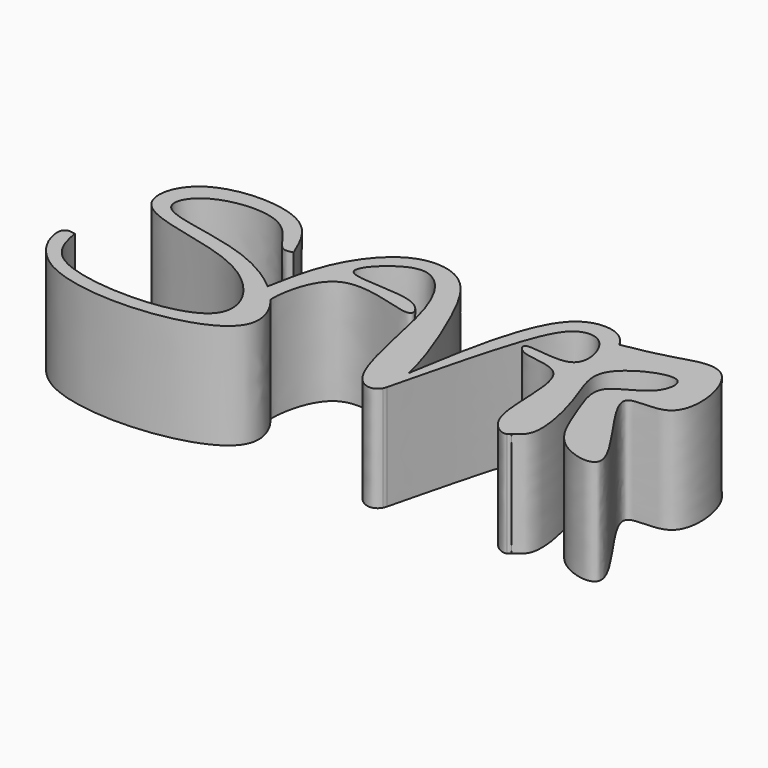
from build123d import *

# Parameters (mm, degrees)
F1_DEPTH = 25.4


# Not quite as in the source:
# - ends of sketch curves that miss each other by under 0.0002 mm in the source are joined


with BuildPart() as f1:
    # F0 (on Top) → F1 (new body)
    with BuildSketch(Plane.XY):
        with BuildLine():
            add(Edge.make_bspline(
                [(-24.6787276119, 32.8070372343), (-25.5273015557, 32.5405150057), (-28.1014851586, 31.7320089754), (-32.90699094, 43.9368654397), (-52.875406472, 41.759288149), (-57.7038976314, 29.1589085216), (-35.7015094106, 29.7052712427), (-22.4863598149, 21.2072316293), (-19.8319724851, 18.9303140968)],
                knots=[0, 0, 0, 0, 0.0470421865, 0.1427043876, 0.2659306317, 0.3432443836, 0.4950399565, 0.5430279559, 0.5430279559, 0.5430279559, 0.5430279559], degree=3))
            add(Edge.make_bspline(
                [(-24.6787276119, 32.8070372343), (-26.5064995292, 37.1770989066), (-30.6352734039, 47.0486787753), (-57.5475208508, 46.96673089), (-62.4266866267, 26.0189740304), (-28.0149183626, 26.4603141136), (-10.52810376, -1.8863198777), (-58.7127529187, -1.6477709858), (-60.8782500601, 8.9999767274), (-61.6968199611, 13.0248842761)],
                knots=[0, 0, 0, 0, 0.1202382283, 0.2716074424, 0.38221019, 0.5584756929, 0.6980251192, 0.8858518243, 1, 1, 1, 1], degree=3))
            add(Edge.make_bspline(
                [(-15.8314434419, 14.8124826193), (-12.8167424406, 10.9820745517), (-8.3770839751, -3.436383487), (-60.1878877743, -8.036598746), (-66.2173758507, 13.782419329), (-62.7256533774, 13.1972916958), (-61.6968199611, 13.0248842761)],
                knots=[0.5706803148, 0.5706803148, 0.5706803148, 0.5706803148, 0.6455092316, 0.8394088149, 0.9526819274, 1, 1, 1, 1], degree=3))
            add(Edge.make_bspline(
                [(-16.0199403512, 15.048879084), (-15.97340642, 14.8563692593), (-15.9033936949, 14.8336509493), (-15.8314434419, 14.8124826193)],
                knots=[0.9896211656, 0.9896211656, 0.9896211656, 0.9896211656, 1, 1, 1, 1], degree=3))
            add(Edge.make_bspline(
                [(-19.8319724851, 18.9303140968), (-18.387658044, 17.6913898312), (-17.0972678041, 16.3826850288), (-16.0199403512, 15.048879084)],
                knots=[0.5430279559, 0.5430279559, 0.5430279559, 0.5430279559, 0.5691393526, 0.5691393526, 0.5691393526, 0.5691393526], degree=3))
        make_face()
        with BuildLine():
            add(Edge.make_bspline(
                [(-19.8319724851, 18.9303140968), (-18.8344760031, 24.2294951854), (-16.8978653598, 34.5465657632), (-6.7743663409, 46.7500210317), (6.8605077442, 45.9638720477), (14.2191273717, 33.5824908681), (21.6696104289, 14.3933148786), (23.0455104144, 7.8380652192)],
                knots=[0, 0, 0, 0, 0.0756121009, 0.147274394, 0.2086812387, 0.2887345767, 0.3572017989, 0.3572017989, 0.3572017989, 0.3572017989], degree=3))
            add(Edge.make_bspline(
                [(-19.8319724851, 18.9303140968), (-18.387658044, 17.6913898312), (-17.0972678041, 16.3826850288), (-16.0199403512, 15.048879084)],
                knots=[0.5430279559, 0.5430279559, 0.5430279559, 0.5430279559, 0.5691393526, 0.5691393526, 0.5691393526, 0.5691393526], degree=3))
            add(Edge.make_bspline(
                [(23.1118220836, 0), (22.177252315, -1.7340239565), (14.5773230299, -1.6966887198), (11.0961627452, 28.9295857186), (3.7256594235, 41.5664043956), (-4.1210514113, 43.3103447304), (-17.5436302823, 30.2403774921), (5.7533981015, 33.779177956), (11.0421016778, 23.3480646444), (-14.612230045, 36.7399787183), (-16.3443080286, 16.3907808564), (-16.0199403512, 15.048879084)],
                knots=[0.393623583, 0.393623583, 0.393623583, 0.393623583, 0.4353913281, 0.5377331001, 0.609740231, 0.6592510214, 0.7193383912, 0.7960567893, 0.8361379212, 0.917274851, 0.9896211656, 0.9896211656, 0.9896211656, 0.9896211656], degree=3))
            add(Edge.make_bspline(
                [(23.4237621025, 0.8001007005), (23.3421922869, 0.5029517859), (23.2386923409, 0.2353982259), (23.1118220836, 0)],
                knots=[0.3879535039, 0.3879535039, 0.3879535039, 0.3879535039, 0.393623583, 0.393623583, 0.393623583, 0.393623583], degree=3))
            add(Edge.make_bspline(
                [(23.0455104144, 7.8380652192), (23.6634889039, 4.8938081328), (23.86615644, 2.4116894523), (23.4237621025, 0.8001007005)],
                knots=[0.3572017989, 0.3572017989, 0.3572017989, 0.3572017989, 0.3879535039, 0.3879535039, 0.3879535039, 0.3879535039], degree=3))
        make_face()
        with BuildLine():
            add(Edge.make_bspline(
                [(-16.0199403512, 15.048879084), (-15.97340642, 14.8563692593), (-15.9033936949, 14.8336509493), (-15.8314434419, 14.8124826193)],
                knots=[0.9896211656, 0.9896211656, 0.9896211656, 0.9896211656, 1, 1, 1, 1], degree=3))
            add(Edge.make_bspline(
                [(-16.0199403512, 15.048879084), (-15.9563619495, 14.9701646226), (-15.8935255947, 14.89136274), (-15.8314434419, 14.8124826193)],
                knots=[0.5691393526, 0.5691393526, 0.5691393526, 0.5691393526, 0.5706803148, 0.5706803148, 0.5706803148, 0.5706803148], degree=3))
        make_face()
        with BuildLine():
            add(Edge.make_bspline(
                [(23.0455104144, 7.8380652192), (24.4324002035, 16.2806044304), (26.8519423128, 31.2653069215), (33.7083031751, 46.5916934343), (43.5702899083, 46.203123325), (46.2558693347, 42.6872189335), (46.7942668802, 41.7043013302)],
                knots=[0, 0, 0, 0, 0.0922168762, 0.1637277559, 0.2200942558, 0.23759776, 0.23759776, 0.23759776, 0.23759776], degree=3))
            add(Edge.make_bspline(
                [(23.0455104144, 7.8380652192), (23.6634889039, 4.8938081328), (23.86615644, 2.4116894523), (23.4237621025, 0.8001007005)],
                knots=[0.3572017989, 0.3572017989, 0.3572017989, 0.3572017989, 0.3879535039, 0.3879535039, 0.3879535039, 0.3879535039], degree=3))
            add(Edge.make_bspline(
                [(53.0788488686, 0), (51.8984399331, -0.5129918214), (44.5848763075, 3.7283170523), (49.1362338719, 28.5544108949), (34.8165799276, 26.4831796905), (31.1780051516, 32.2004713219), (48.3201512021, 26.7229973916), (44.5678259808, 41.4874538831), (36.376462422, 42.3677304518), (30.6036182602, 31.4239322121), (24.2879136847, 3.9486155232), (23.4239237173, 0.8006904499), (23.4237621025, 0.8001007005)],
                knots=[0.4289942329, 0.4289942329, 0.4289942329, 0.4289942329, 0.4767021069, 0.5614775501, 0.6211663392, 0.6508244204, 0.7128544037, 0.7693222766, 0.8141842446, 0.8799646816, 0.9827832344, 0.9828025139, 0.9828025139, 0.9828025139, 0.9828025139], degree=3))
            add(Edge.make_bspline(
                [(53.6664426327, 0.63326415), (53.3590889397, 0.4114939862), (53.2189711295, 0.2057502607), (53.0788488686, 0)],
                knots=[0.9808770796, 0.9808770796, 0.9808770796, 0.9808770796, 1, 1, 1, 1], degree=3))
            add(Edge.make_bspline(
                [(46.7942668802, 41.7043013302), (48.6032933073, 38.4016786955), (50.3660101546, 25.8827463669), (53.5382364777, 8.1673975806), (54.0836898285, 1.5815416662), (53.6664426327, 0.63326415)],
                knots=[0.23759776, 0.23759776, 0.23759776, 0.23759776, 0.2964098812, 0.385024933, 0.4183512362, 0.4183512362, 0.4183512362, 0.4183512362], degree=3))
        make_face()
        with BuildLine():
            add(Edge.make_bspline(
                [(23.4237621025, 0.8001007005), (23.3421922869, 0.5029517859), (23.2386923409, 0.2353982259), (23.1118220836, 0)],
                knots=[0.3879535039, 0.3879535039, 0.3879535039, 0.3879535039, 0.393623583, 0.393623583, 0.393623583, 0.393623583], degree=3))
            add(Edge.make_bspline(
                [(23.4237621025, 0.8001007005), (23.2793710251, 0.2741020489), (23.2183930531, 0.1282770233), (23.1118220836, 0)],
                knots=[0.9828025139, 0.9828025139, 0.9828025139, 0.9828025139, 1, 1, 1, 1], degree=3))
        make_face()
        with BuildLine():
            add(Edge.make_bspline(
                [(46.7942668802, 41.7043013302), (50.3848090207, 42.3444269721), (57.5784609028, 43.6240432253), (71.8688709785, 49.2296239678), (76.4397987852, 22.0429179865), (52.8460197012, 29.7031437768), (81.6110286462, -1.4014680593), (62.3170902407, 1.8533546119), (58.0399247272, 14.7977347688), (52.7378625165, 26.9256595732), (65.0537492941, 29.5782405699), (66.4716848994, 40.8014290246), (47.9292406475, 32.4847086055), (54.1956479046, 20.498618098), (58.4414610746, 2.7191685618), (54.2851661425, 1.0797023003), (53.6664426327, 0.63326415)],
                knots=[0, 0, 0, 0, 0.0696168426, 0.139557473, 0.2251970613, 0.2894080935, 0.3920456325, 0.4510893761, 0.5301929119, 0.5963398453, 0.6612406867, 0.7111688526, 0.7855380932, 0.8574622076, 0.9423813637, 0.9808770796, 0.9808770796, 0.9808770796, 0.9808770796], degree=3))
            add(Edge.make_bspline(
                [(46.7942668802, 41.7043013302), (48.6032933073, 38.4016786955), (50.3660101546, 25.8827463669), (53.5382364777, 8.1673975806), (54.0836898285, 1.5815416662), (53.6664426327, 0.63326415)],
                knots=[0.23759776, 0.23759776, 0.23759776, 0.23759776, 0.2964098812, 0.385024933, 0.4183512362, 0.4183512362, 0.4183512362, 0.4183512362], degree=3))
        make_face()
        with BuildLine():
            add(Edge.make_bspline(
                [(53.6664426327, 0.63326415), (53.3590889397, 0.4114939862), (53.2189711295, 0.2057502607), (53.0788488686, 0)],
                knots=[0.9808770796, 0.9808770796, 0.9808770796, 0.9808770796, 1, 1, 1, 1], degree=3))
            add(Edge.make_bspline(
                [(53.6664426327, 0.63326415), (53.5331917132, 0.3304248446), (53.342182515, 0.1144417014), (53.0788488686, 0)],
                knots=[0.4183512362, 0.4183512362, 0.4183512362, 0.4183512362, 0.4289942329, 0.4289942329, 0.4289942329, 0.4289942329], degree=3))
        make_face()
    extrude(amount=F1_DEPTH)


solid = f1.part
